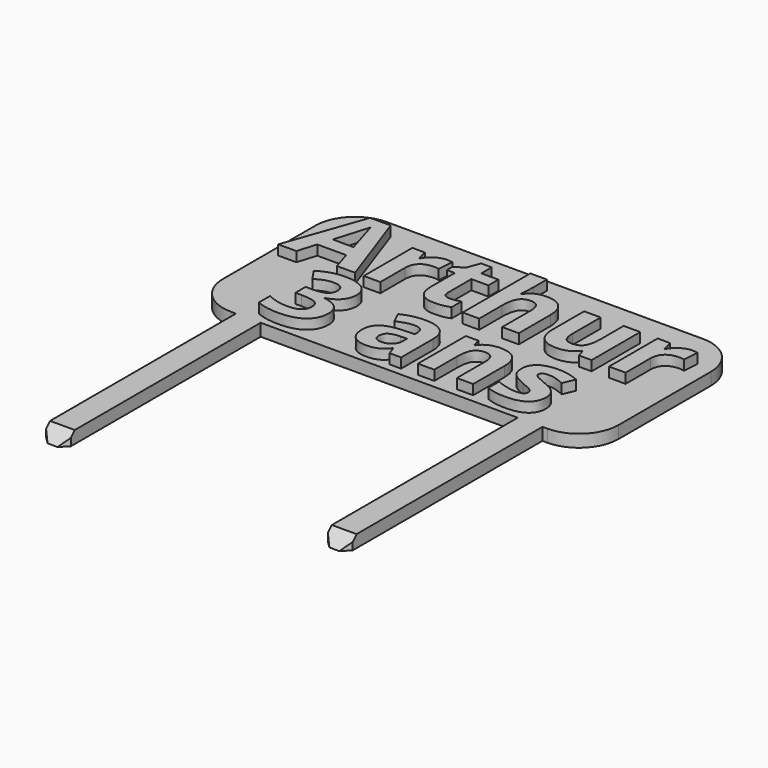
from build123d import *

# Parameters (mm, degrees)
F0_W           = 80
F0_H           = 39.3282976002
F1_DEPTH       = 2.5
F2_TEXT_SIZE   = 22.5227982617
F2_TEXT_SIZE_2 = 22.1674021167
F3_DEPTH       = 2
F4_W           = 5
F4_H           = 50
F5_DEPTH       = 2.5
F6_R           = 8
F7_SIZE        = 2
F8_T1_DEPTH    = 16.4300979278
F8_T3_DEPTH    = 16.4300979278


# Not quite as in the source:
# - a fillet or chamfer that OpenCascade refuses, or shapes differently, is made with other operations: its cross-section is extruded or revolved along the edge and cut away or added
# - Text() gives the source's letters only with a copy of the font that has no kerning and outlines rounded to 1/6400 em; it was checked with that copy


with BuildPart() as f1:
    # F0 (on Top) → F1 (new body)
    with BuildSketch(Plane.XY):
        Rectangle(F0_W, F0_H)
    extrude(amount=F1_DEPTH)

    # F2 (on face) → F3 (join)
    with BuildSketch(Plane.XY.offset(2.5)):
        with Locations((-38.1814218345, 0)):
            Text('Arthur', F2_TEXT_SIZE, font='Open Sans', font_style=FontStyle.BOLD, text_align=(TextAlign.LEFT, TextAlign.BOTTOM))
        with Locations((-28.9925374091, -18.0762012798)):
            Text('3 ans', F2_TEXT_SIZE_2, font='Open Sans', font_style=FontStyle.BOLD, text_align=(TextAlign.LEFT, TextAlign.BOTTOM))
    extrude(amount=F3_DEPTH)

    # F4 (on Top) → F5 (join)
    with BuildSketch(Plane.XY):
        with Locations((-28.5, -44.6641488001)):
            Rectangle(F4_W, F4_H)
        with Locations((28.5, -44.6641488001)):
            Rectangle(F4_W, F4_H)
    extrude(amount=F5_DEPTH)

    # F6
    f6_edges = [f1.edges().sort_by_distance(p)[0] for p in [
        (40, -19.664149, 1.25),
        (40, 19.664149, 1.25),
        (-40, -19.664149, 1.25),
        (-40, 19.664149, 1.25),
    ]]
    fillet(f6_edges, radius=F6_R)

    # F7
    f7_edges = [f1.edges().sort_by_distance(p)[0] for p in [
        (-31, -69.664149, 1.25),
        (-26, -69.664149, 1.25),
        (26, -69.664149, 1.25),
        (31, -69.664149, 1.25),
    ]]
    chamfer(f7_edges, length=F7_SIZE)

    # F8: chamfer of 3 on 2 edges, made by hand

    # F8_s2 → F8_t1 (cut)
    with BuildSketch(Plane.YZ.offset(-36.7150489639)):
        Polygon((-69.6641488001, -0.5), (-66.6641488001, 2.5), (-69.6641488001, 2.5), align=None)
    extrude(amount=F8_T1_DEPTH, mode=Mode.SUBTRACT)

    # F8_s4 → F8_t3 (cut)
    with BuildSketch(Plane.YZ.offset(20.2849510361)):
        Polygon((-69.6641488001, -0.5), (-66.6641488001, 2.5), (-69.6641488001, 2.5), align=None)
    extrude(amount=F8_T3_DEPTH, mode=Mode.SUBTRACT)


solid = f1.part
